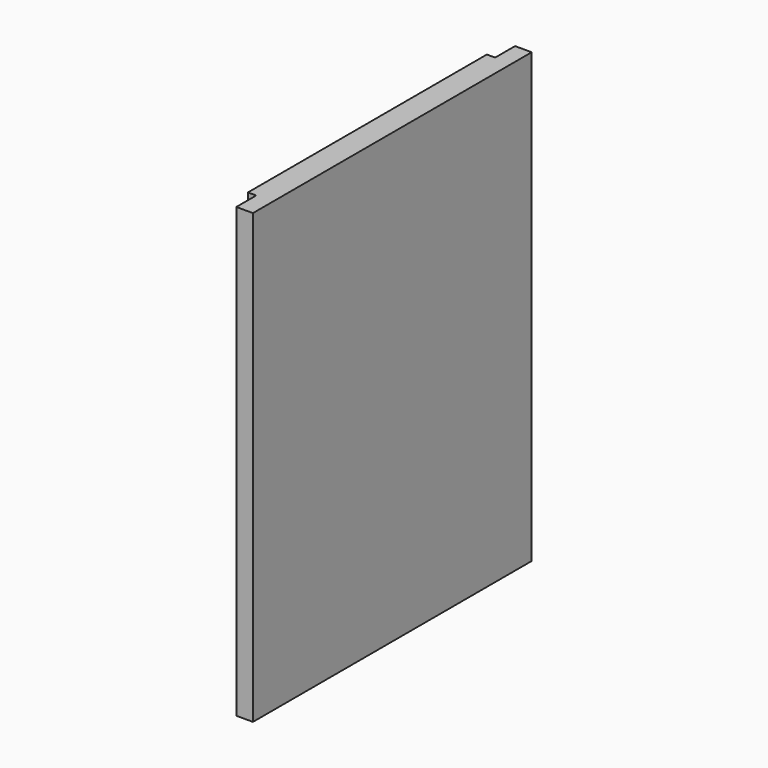
from build123d import *

# Parameters (mm, degrees)
F0_W     = 88.9
F0_H     = 114.3
F1_DEPTH = 4.2418
F2_W     = 76.2
F2_H     = 114.3
F3_DEPTH = 2.11582


# Not quite as in the source:
# - a feature names something its author has since deleted; it is built from what else it names


with BuildPart() as f1:
    # F0 (on Right) → F1 (new body)
    with BuildSketch(Plane.YZ):
        with Locations((44.45, 57.15)):
            Rectangle(F0_W, F0_H)
    extrude(amount=F1_DEPTH)

    # F2 (on Right) → F3 (join)
    with BuildSketch(Plane.YZ):
        with Locations((44.45, 57.15)):
            Rectangle(F2_W, F2_H)
    extrude(amount=-F3_DEPTH)


solid = f1.part
